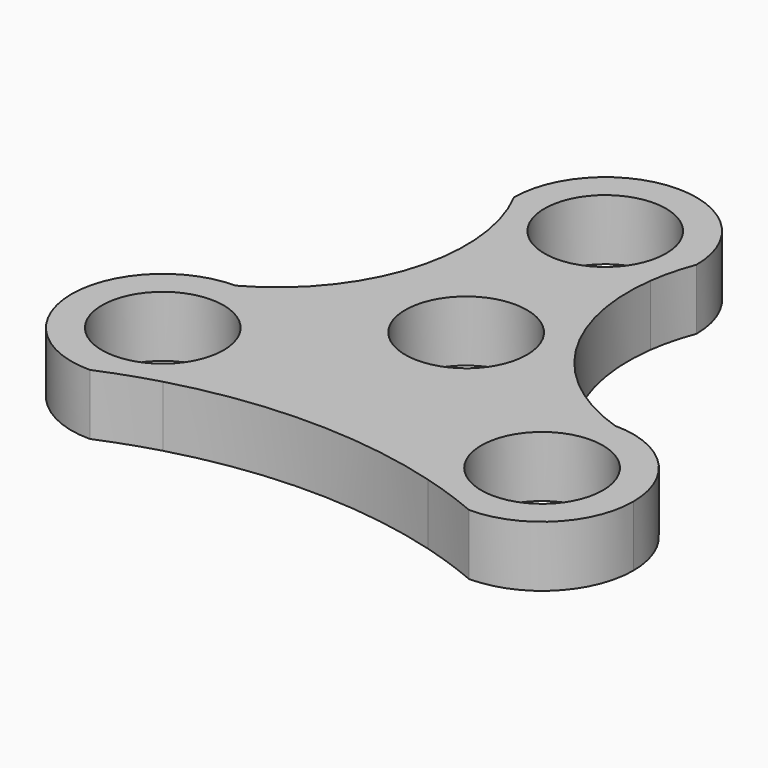
from build123d import *

# Parameters (mm, degrees)
F1_DEPTH = 25.4
F2_R     = 6.35
F3_DEPTH = 25.401
F4_DEPTH = 19.05
F5_R     = 6.35
F6_DEPTH = 6.351


with BuildPart() as f1:
    # F0 (on Top) → F1 (new body)
    with BuildSketch(Plane.XY):
        with BuildLine():
            ThreePointArc((-11.9960894898, 7.8287454173), (-22.8140252531, 16.2307401146), (-25.7390544228, 29.6122741608))
            ThreePointArc((-25.7390544228, 29.6122741608), (-33.3767507176, 24.6782589704), (-41.673253936, 28.3994073062))
            ThreePointArc((-41.673253936, 28.3994073062), (-43.3440087931, 16.5245060033), (-51.6016386333, 7.8287454173))
            ThreePointArc((-51.6016386333, 7.8287454173), (-44.8664465425, 5.0389375081), (-42.0766386333, -1.6962545827))
            ThreePointArc((-42.0766386333, -1.6962545827), (-43.013362785, -5.8153737791), (-45.6392933218, -9.1243137765))
            ThreePointArc((-45.6392933218, -9.1243137765), (-31.7988640615, -7.20255554), (-17.9584348012, -9.1243137765))
            ThreePointArc((-17.9584348012, -9.1243137765), (-20.9815746971, 1.463916392), (-11.9960894898, 7.8287454173))
        make_face()
        with BuildLine():
            ThreePointArc((-42.0766386333, -1.6962545827), (-44.8664465425, 5.0389375081), (-51.6016386333, 7.8287454173))
            ThreePointArc((-51.6016386333, 7.8287454173), (-61.1266386333, -1.6962545827), (-51.6016386333, -11.2212545827))
            ThreePointArc((-51.6016386333, -11.2212545827), (-48.6531092599, -10.0799677677), (-45.6392933218, -9.1243137765))
            ThreePointArc((-45.6392933218, -9.1243137765), (-43.013362785, -5.8153737791), (-42.0766386333, -1.6962545827))
        make_face()
        with BuildLine():
            ThreePointArc((-2.4710894898, -1.6962545827), (-5.260897399, 5.0389375081), (-11.9960894898, 7.8287454173))
            ThreePointArc((-11.9960894898, 7.8287454173), (-20.9815746971, 1.463916392), (-17.9584348012, -9.1243137765))
            ThreePointArc((-17.9584348012, -9.1243137765), (-14.9446188632, -10.0799677677), (-11.9960894898, -11.2212545827))
            ThreePointArc((-11.9960894898, -11.2212545827), (-5.260897399, -8.4314466735), (-2.4710894898, -1.6962545827))
        make_face()
        with BuildLine():
            ThreePointArc((-25.7390544228, 29.6122741608), (-25.2909601874, 31.9282439717), (-24.5746759409, 34.175785181))
            ThreePointArc((-24.5746759409, 34.175785181), (-34.0996759409, 43.700785181), (-43.6246759409, 34.175785181))
            ThreePointArc((-43.6246759409, 34.175785181), (-42.4236958583, 31.3636984394), (-41.673253936, 28.3994073062))
            ThreePointArc((-41.673253936, 28.3994073062), (-33.3767507176, 24.6782589704), (-25.7390544228, 29.6122741608))
        make_face()
    extrude(amount=F1_DEPTH)

    # F2 (on face) → F3 (cut, through all)
    with BuildSketch(Plane.XY.offset(25.4)):
        with Locations((-51.6016386333, -1.6962545827)):
            Circle(F2_R)
        with Locations((-11.9960894898, -1.6962545827)):
            Circle(F2_R)
        with Locations((-34.0996759409, 34.175785181)):
            Circle(F2_R)
    extrude(amount=-F3_DEPTH, mode=Mode.SUBTRACT)

    # F4 (cut): a face of the model
    f4_faces = [f1.faces().sort_by_distance(p)[0] for p in [
        (-32.4383450301, 9.0422986836, 25.4),
    ]]
    extrude(f4_faces, amount=-F4_DEPTH, mode=Mode.SUBTRACT)

    # F5 (on face) → F6 (cut, through all)
    with BuildSketch(Plane.XY.offset(6.35)):
        with Locations((-31.778564126, 13.1174343201)):
            Circle(F5_R)
    extrude(amount=-F6_DEPTH, mode=Mode.SUBTRACT)


solid = f1.part
